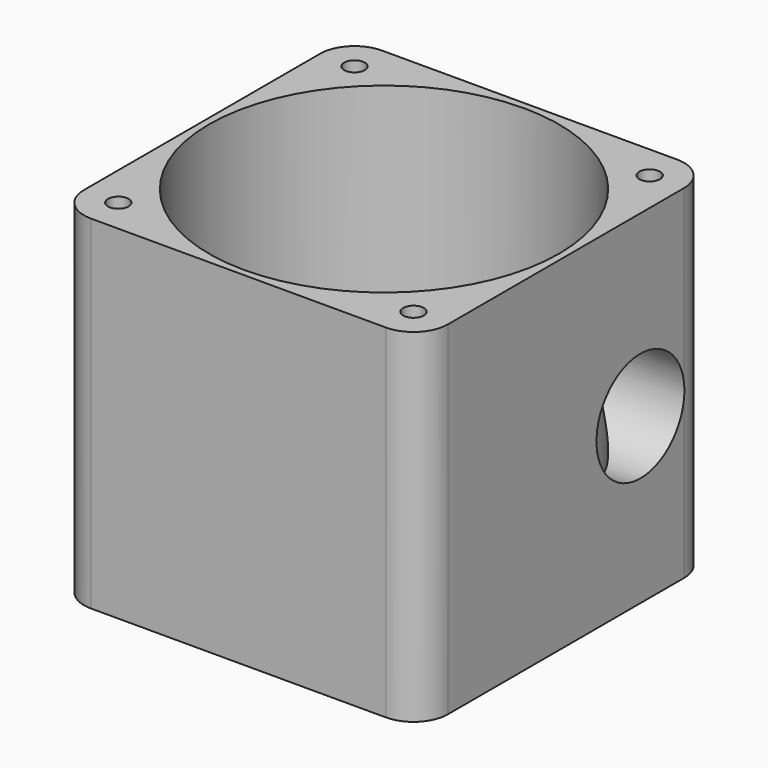
from build123d import *

# Parameters (mm, degrees)
F0_R     = 25.5
F1_DEPTH = 50
F0_R_2   = 11.625
F2_DEPTH = 9
F4_R     = 8
F5_DEPTH = 15
F8_D     = 3
F8_DEPTH = 8
F8_TIP   = 0.9012909285


with BuildPart() as f1:
    # F0 (on Top) → F1 (new body)
    with BuildSketch(Plane.XY):
        with BuildLine():
            Line((21.5, 26.5), (-21.5, 26.5))
            ThreePointArc((-21.5, 26.5), (-25.0355339059, 25.0355339059), (-26.5, 21.5))
            Line((-26.5, 21.5), (-26.5, -21.5))
            ThreePointArc((-26.5, -21.5), (-25.0355339059, -25.0355339059), (-21.5, -26.5))
            Line((-21.5, -26.5), (21.5, -26.5))
            ThreePointArc((21.5, -26.5), (25.0355339059, -25.0355339059), (26.5, -21.5))
            Line((26.5, -21.5), (26.5, 21.5))
            ThreePointArc((26.5, 21.5), (25.0355339059, 25.0355339059), (21.5, 26.5))
        make_face()
        Circle(F0_R, mode=Mode.SUBTRACT)
    extrude(amount=F1_DEPTH)

    # F0 (on Top) → F2 (join)
    with BuildSketch(Plane.XY):
        Circle(F0_R)
        Circle(F0_R_2, mode=Mode.SUBTRACT)
    extrude(amount=F2_DEPTH)

    # F4 (on offset) → F5 (cut)
    with BuildSketch(Plane.YZ.offset(26.5)):
        with Locations((13.5627460668, 24)):
            Circle(F4_R)
    extrude(amount=-F5_DEPTH, mode=Mode.SUBTRACT)

    # F8
    with Locations(Plane.XY.offset(50)):
        with Locations((-21.5, 21.5), (21.5, 21.5), (21.5, -21.5), (-21.5, -21.5)):
            Hole(F8_D / 2, depth=F8_DEPTH)
            with Locations((0, 0, -(F8_DEPTH + F8_TIP / 2))):  # 118° drill point
                Cone(0, F8_D / 2, F8_TIP, mode=Mode.SUBTRACT)


solid = f1.part
